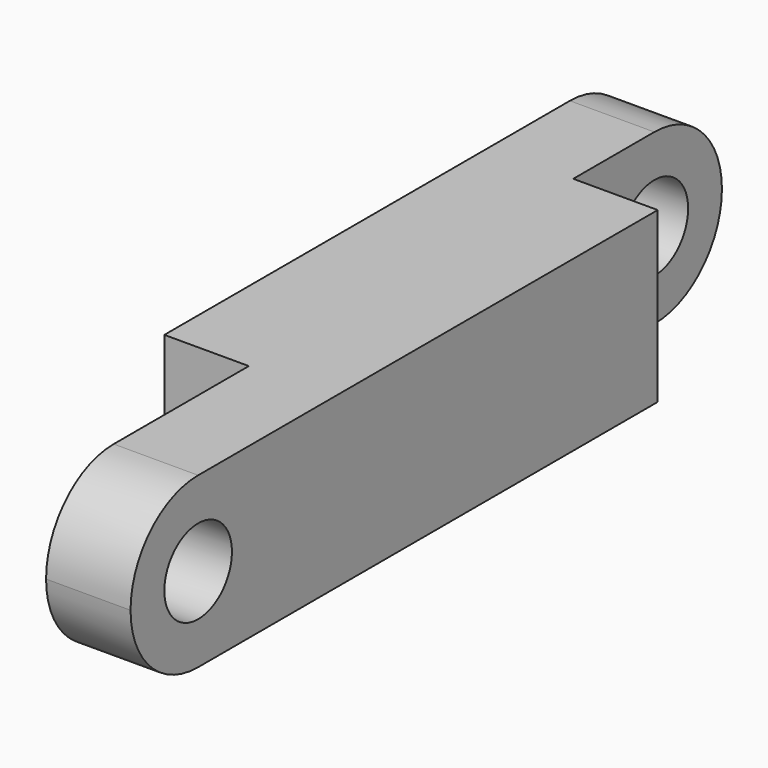
from build123d import *

# Parameters (mm, degrees)
F0_W     = 20
F0_H     = 20
F1_DEPTH = 100
F2_R     = 5
F3_DEPTH = 20.001
F4_R     = 5
F5_DEPTH = 20.001
F6_W     = 22
F6_H     = 20
F6_R     = 5
F7_DEPTH = 10
F8_W     = 30
F8_H     = 20
F8_R     = 5
F9_DEPTH = 10
F10_R    = 9.99999


# Not quite as in the source:
# - a fillet or chamfer is up to 0.001 mm smaller than in the source, because OpenCascade refuses the exact size


with BuildPart() as f1:
    # F0 (on Front) → F1 (new body)
    with BuildSketch(Plane.XZ):
        Rectangle(F0_W, F0_H)
    extrude(amount=F1_DEPTH)

    # F2 (on face) → F3 (cut, through all)
    with BuildSketch(Plane.YZ.offset(10)):
        with Locations((-90, 0)):
            Circle(F2_R)
    extrude(amount=-F3_DEPTH, mode=Mode.SUBTRACT)

    # F4 (on face) → F5 (cut, through all)
    with BuildSketch(Plane.YZ.offset(10)):
        with Locations((-10, 0)):
            Circle(F4_R)
    extrude(amount=-F5_DEPTH, mode=Mode.SUBTRACT)

    # F6 (on face) → F7 (cut)
    with BuildSketch(Plane.YZ.offset(10)):
        with Locations((-11, 0)):
            Rectangle(F6_W, F6_H)
        with Locations((-10, 0)):
            Circle(F6_R, mode=Mode.SUBTRACT)
    extrude(amount=-F7_DEPTH, mode=Mode.SUBTRACT)

    # F8 (on face) → F9 (cut)
    with BuildSketch(Plane(origin=(-10, 0, 0), x_dir=(0, -1, 0), z_dir=(-1, 0, 0))):
        with Locations((85, 0)):
            Rectangle(F8_W, F8_H)
        with Locations((90, 0)):
            Circle(F8_R, mode=Mode.SUBTRACT)
    extrude(amount=-F9_DEPTH, mode=Mode.SUBTRACT)

    # F10 (radius 10 in the source; OpenCascade refuses exactly that, so slightly less here)
    f10_edges = [f1.edges().sort_by_distance(p)[0] for p in [
        (5, -100, 10),
        (5, -100, -10),
        (-5, 0, -10),
        (-5, 0, 10),
    ]]
    fillet(f10_edges, radius=F10_R)


solid = f1.part
